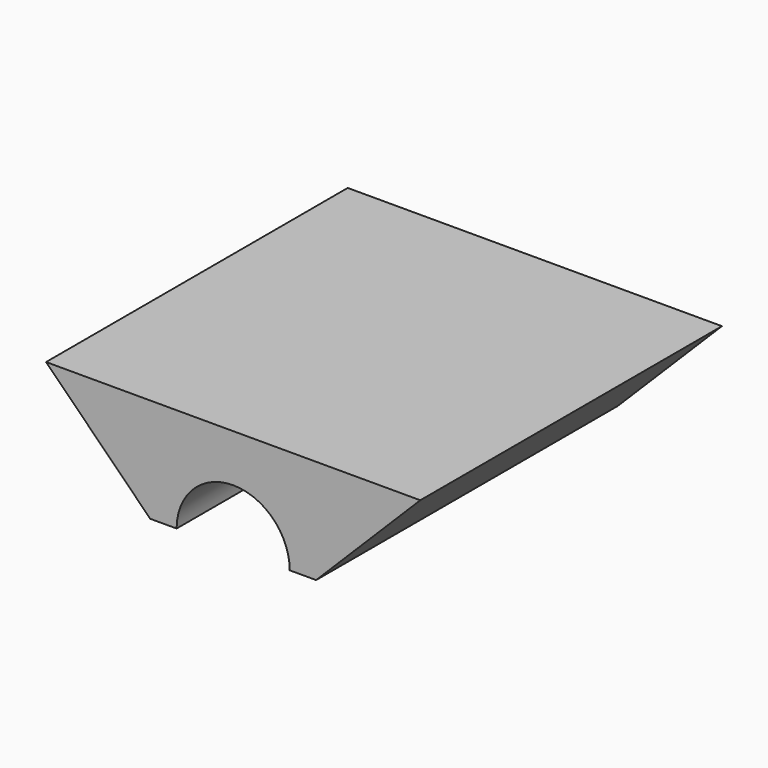
from build123d import *

# Parameters (mm, degrees)
F2_DEPTH    = 63.5
F3_T1_DEPTH = 154.9490470521


# Not quite as in the source:
# - a fillet or chamfer that OpenCascade refuses, or shapes differently, is made with other operations: its cross-section is extruded or revolved along the edge and cut away or added


with BuildPart() as f2:
    # F1 (on face) → F2 (new body)
    with BuildSketch(Plane.XZ):
        with BuildLine():
            ThreePointArc((-9.525, 0), (0, 9.525), (9.525, 0))
            Line((9.525, 0), (17.9719245062, 0))
            Line((17.9719245062, 0), (31.75, 0))
            Line((31.75, 0), (31.75, 17.5402989774))
            Line((31.75, 17.5402989774), (-31.75, 17.5402989774))
            Line((-31.75, 17.5402989774), (-31.75, 0))
            Line((-31.75, 0), (-17.9475410922, 0))
            Line((-17.9475410922, 0), (-9.525, 0))
        make_face()
    extrude(amount=F2_DEPTH)

    # F3: chamfer of 17.78 on 2 edges, made by hand

    # F3_s2 → F3_t1 (cut)
    with BuildSketch(Plane.XZ.offset(-45.724523526)):
        Polygon((-31.75, 17.78), (-13.97, 0), (-31.75, 0), align=None)
        Polygon((31.75, 17.78), (13.97, 0), (31.75, 0), align=None)
    extrude(amount=F3_T1_DEPTH, mode=Mode.SUBTRACT)


solid = f2.part
